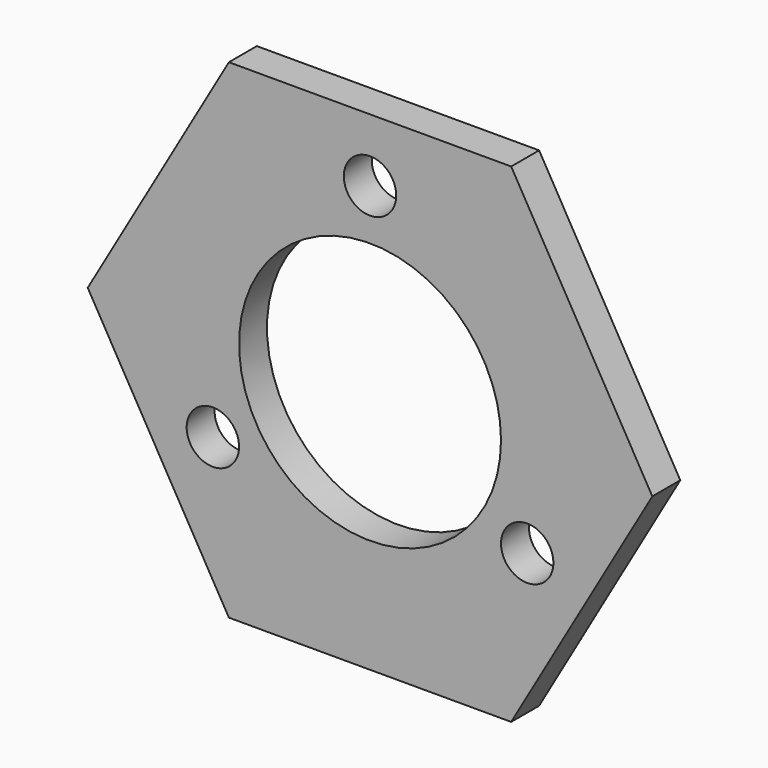
from build123d import *

# Parameters (mm, degrees)
F0_R     = 4.7625
F0_R_2   = 23.8125
F1_DEPTH = 6.35


# Not quite as in the source:
# - the program builds the solid bodies; features that only make, move or delete a surface that nothing else refers to are left out


with BuildPart() as f1:
    # F0 (on Front) → F1 (new body)
    with BuildSketch(Plane.XZ):
        Polygon((-25.6632194655, 44.45), (-51.326438931, 0), (-25.6632194655, -44.45), (25.6632194655, -44.45), (51.326438931, 0), (25.6632194655, 44.45), align=None)
        with Locations((-28.5741617877, -16.4973)):
            Circle(F0_R, mode=Mode.SUBTRACT)
        with Locations((28.5741617877, -16.4973)):
            Circle(F0_R, mode=Mode.SUBTRACT)
        Circle(F0_R_2, mode=Mode.SUBTRACT)
        with Locations((0, 32.9946)):
            Circle(F0_R, mode=Mode.SUBTRACT)
    extrude(amount=-F1_DEPTH)


solid = f1.part
